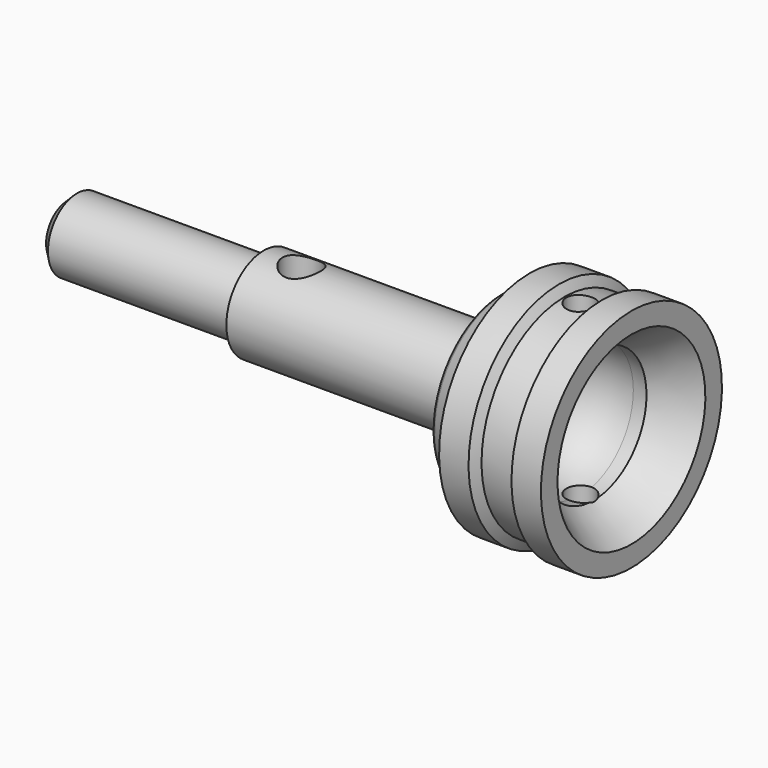
from build123d import *

# Parameters (mm, degrees)
F8_R          = 0.75
F8_R_2        = 1
F9_DEPTH      = 6.001
F9_DEPTH_BACK = 6.001
F11_SIZE      = 0.5
F12_R         = 0.5
F13_R         = 0.3


# Not quite as in the source:
# - a fillet or chamfer that OpenCascade refuses, or shapes differently, is made with other operations: its cross-section is extruded or revolved along the edge and cut away or added


with BuildPart() as f4:
    # F3 (on Front) → F4 (revolve)
    with BuildSketch(Plane.XZ):
        with BuildLine():
            Line((2.7, 6), (-2.7, 6))
            Line((-2.7, 6), (-2.7, 5.3))
            Line((-2.7, 5.3), (-4.3, 4.5))
            Line((-4.3, 4.5), (-4.3, 2.775))
            ThreePointArc((-4.3, 2.775), (-4.3878679656, 2.5628679656), (-4.6, 2.475))
            Line((-4.6, 2.475), (-16.8, 2.475))
            Line((-16.8, 2.475), (-16.8, 1.925))
            Line((-16.8, 1.925), (-27.2, 1.925))
            Line((-27.2, 1.925), (-27.2, 0))
            Line((-27.2, 0), (2.7, 0))
            Line((2.7, 0), (2.7, 6))
        make_face()
    revolve(axis=Axis((0, 0, 0), (1, 0, 0)))

    # F2 (on Front) → F5 (revolve, cut)
    with BuildSketch(Plane.XZ):
        with BuildLine():
            Line((5, 3.5), (0, 3.5))
            ThreePointArc((0, 3.5), (-2.4748737342, 2.4748737342), (-3.5, 0))
            Line((-3.5, 0), (5, 0))
            Line((5, 0), (5, 3.5))
        make_face()
    revolve(axis=Axis((0, 0, 0), (1, 0, 0)), mode=Mode.SUBTRACT)

    # F6 (on Front) → F7 (revolve, cut)
    with BuildSketch(Plane.XZ):
        Polygon((1.1386751346, 6), (-1.1386751346, 6), (-0.85, 5.5), (0.85, 5.5), align=None)
    revolve(axis=Axis((0, 0, 0), (1, 0, 0)), mode=Mode.SUBTRACT)

    # F8 (on Top) → F9 (cut, two sides)
    with BuildSketch(Plane.XY) as f9_sk:
        Circle(F8_R)
        with Locations((-14.8, 0)):
            Circle(F8_R_2)
    extrude(amount=-F9_DEPTH, mode=Mode.SUBTRACT)
    extrude(f9_sk.sketch, amount=F9_DEPTH_BACK, mode=Mode.SUBTRACT)

    # F10: chamfer of 2 x 1.4004150764 on 1 edges, made by hand

    # F10_s1 → F10_t2 (revolve, cut)
    with BuildSketch(Plane.XZ):
        Polygon((2.7, 4.9004150764), (0.7, 3.5), (2.7, 3.5), align=None)
    revolve(axis=Axis((2.7, 0, 0), (-1, 0, 0)), mode=Mode.SUBTRACT)

    # F11
    f11_edges = [f4.edges().sort_by_distance(p)[0] for p in [
        (-27.2, 0, -1.925),
    ]]
    chamfer(f11_edges, length=F11_SIZE)

    # F12
    f12_edges = [f4.edges().sort_by_distance(p)[0] for p in [
        (-4.3, 0, -4.5),
        (-2.7, 0, -5.3),
    ]]
    fillet(f12_edges, radius=F12_R)

    # F13
    f13_edges = [f4.edges().sort_by_distance(p)[0] for p in [
        (-16.8, 0, -1.925),
    ]]
    fillet(f13_edges, radius=F13_R)


solid = f4.part
